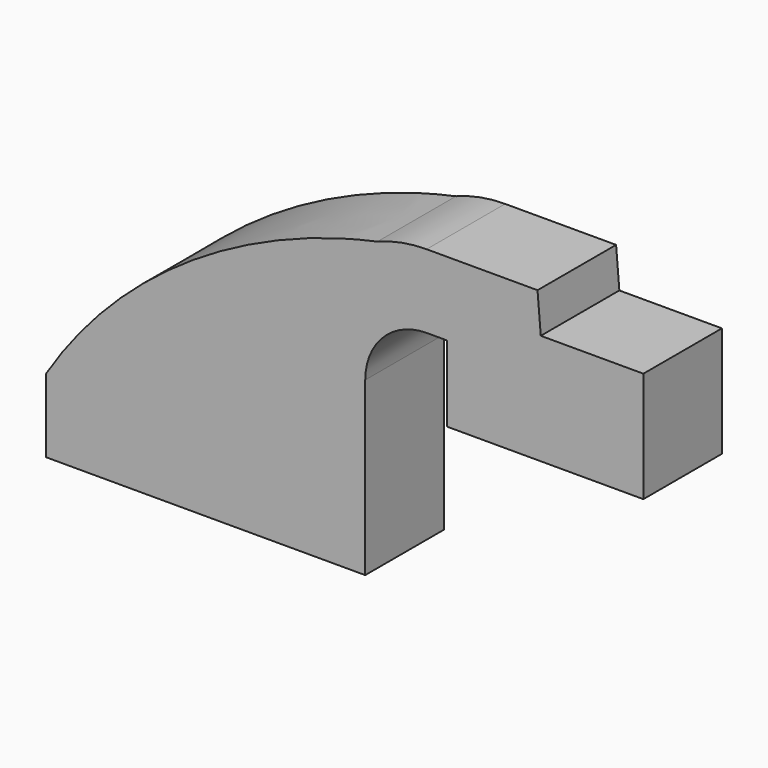
from build123d import *

# Parameters (mm, degrees)
F1_DEPTH = 25.4


with BuildPart() as f1:
    # F0 (on Front) → F1 (new body)
    with BuildSketch(Plane.XZ):
        with BuildLine():
            add(Edge.make_bspline(
                [(-41.275, 9.525), (-22.0747437676, 40.2046527133), (10.3334958868, 60.2024181647), (44.4254317337, 67.4494675196)],
                knots=[0, 0, 0, 0, 100.1940888091, 100.1940888091, 100.1940888091, 100.1940888091], degree=3))
            Line((-41.275, 9.525), (22.225, 9.525))
            Line((22.225, 9.5250000022), (22.225, 34.925))
            ThreePointArc((22.225, 34.925), (28.3041929243, 54.6144651819), (44.4254317337, 67.4494675196))
        make_face()
        Polygon((22.225, 9.525), (-41.275, 9.525), (-41.275, -9.525), (41.275, -9.525), (41.275, 9.525), align=None)
        with BuildLine():
            Line((22.225, 34.925), (22.225, 9.5250000022))
            Line((22.225, 9.525), (41.275, 9.525))
            Line((41.275, 9.525), (41.275, 34.925))
            ThreePointArc((41.275, 34.925), (45.9246798487, 46.1503201513), (57.15, 50.8))
            Line((57.15, 50.8), (62.4140998637, 50.8))
            Line((62.4140998637, 50.8), (62.4140998637, 59.7440389732))
            Line((62.4140998637, 59.7440389732), (86.6818488397, 59.7440389732))
            Line((86.6818488397, 59.7440389732), (85.8401209116, 69.85))
            Line((85.8401209116, 69.85), (59.9131250273, 69.85))
            add(Edge.make_bspline(
                [(44.4254317337, 67.4494675196), (49.5629070715, 68.5415597229), (54.7386173045, 69.3440971379), (59.9131250273, 69.85)],
                knots=[100.1940888091, 100.1940888091, 100.1940888091, 100.1940888091, 115.2928107637, 115.2928107637, 115.2928107637, 115.2928107637], degree=3))
            ThreePointArc((44.4254317337, 67.4494675196), (28.3041929243, 54.6144651819), (22.225, 34.925))
        make_face()
        with BuildLine():
            ThreePointArc((57.15, 69.85), (50.675488556, 69.2446201401), (44.4254317337, 67.4494675196))
            add(Edge.make_bspline(
                [(44.4254317337, 67.4494675196), (49.5629070715, 68.5415597229), (54.7386173045, 69.3440971379), (59.9131250273, 69.85)],
                knots=[100.1940888091, 100.1940888091, 100.1940888091, 100.1940888091, 115.2928107637, 115.2928107637, 115.2928107637, 115.2928107637], degree=3))
            Line((59.9131250273, 69.85), (57.15, 69.85))
        make_face()
        Polygon((87.4268, 50.8), (86.6818488397, 59.7440389732), (62.4140998637, 59.7440389732), (62.4140998637, 50.8), align=None)
        Polygon((113.2140998637, 59.7440389732), (86.6818488397, 59.7440389732), (87.4268, 50.8), (62.4140998637, 50.8), (62.4140998637, 31.1690389732), (113.2140998637, 31.1690389732), align=None)
    extrude(amount=F1_DEPTH)


solid = f1.part
